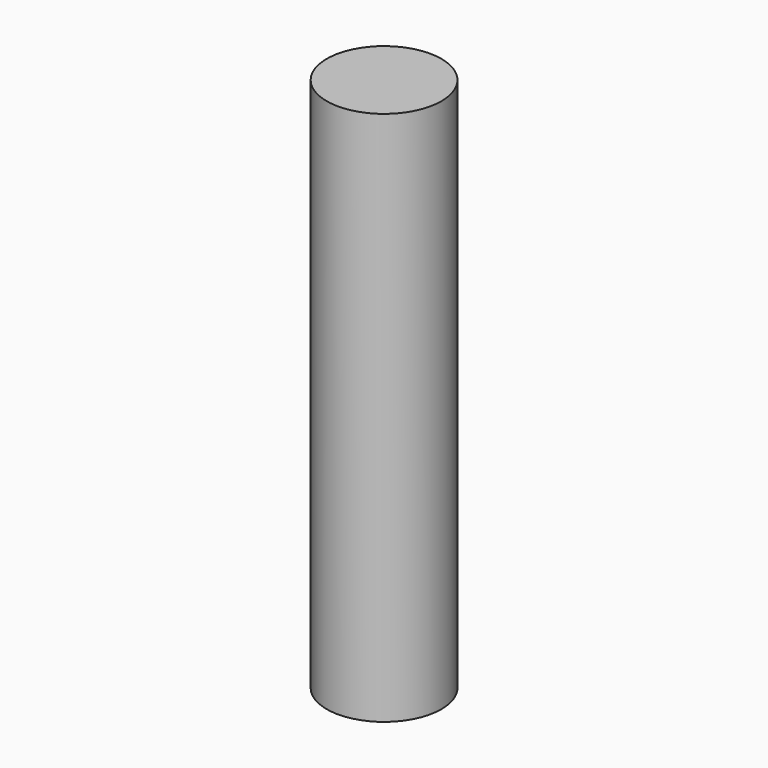
from build123d import *

# Parameters (mm, degrees)
F0_R     = 0.75
F1_DEPTH = 7


# Not quite as in the source:
# - a feature names something its author has since deleted; it is built from what else it names


with BuildPart() as f1:
    # F0 (on Top) → F1 (new body)
    with BuildSketch(Plane.XY):
        with Locations((-13.2808377966, 7.6941782609)):
            Circle(F0_R)
    extrude(amount=F1_DEPTH)


solid = f1.part
